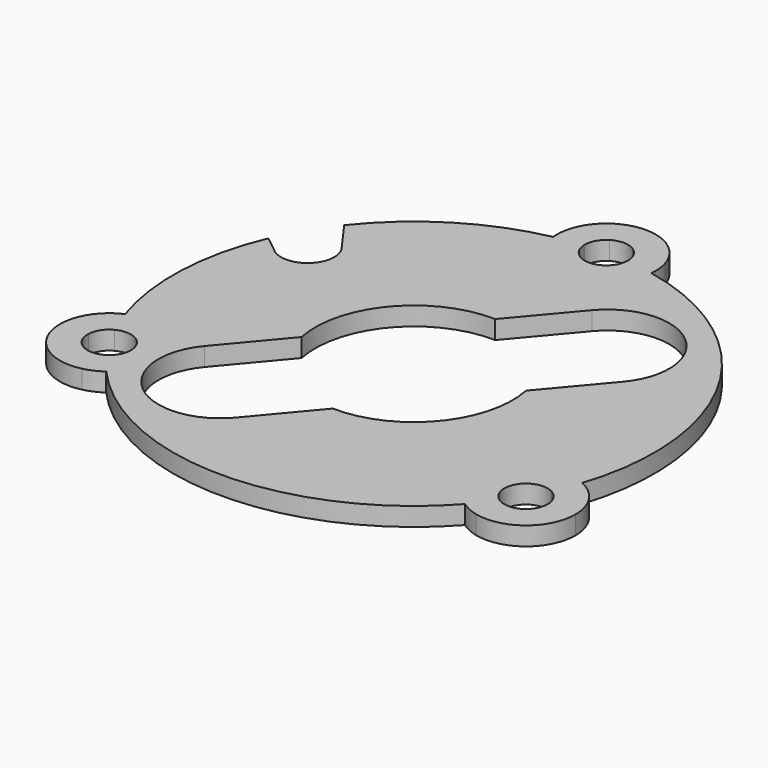
from build123d import *

# Parameters (mm, degrees)
F1_DEPTH = 1.5


# Not quite as in the source:
# - a feature names something its author has since deleted; it is built from what else it names


with BuildPart() as f1:
    # F0 (on Top) → F1 (new body)
    with BuildSketch(Plane.XY):
        with BuildLine():
            Line((-16.6795244343, 6.6792241971), (-17.9256127972, 7.6760931368))
            ThreePointArc((-17.9256127972, 7.6760931368), (-19.4817711686, 0.8429662711), (-18.5216556944, -6.0990384764))
            ThreePointArc((-18.5216556944, -6.0990384764), (-18.1379825879, -7.1598594707), (-17.6936088333, -8.1967192494))
            ThreePointArc((-17.6936088333, -8.1967192494), (-15.9787045712, -8.2544735786), (-15.1374953738, -9.75))
            ThreePointArc((-15.1374953738, -9.75), (-15.3526962413, -10.5907684717), (-15.9453715143, -11.2247551096))
            ThreePointArc((-15.9453715143, -11.2247551096), (-15.2696114831, -12.1280239592), (-14.5427501065, -12.9907051133))
            ThreePointArc((-14.5427501065, -12.9907051133), (0, -19.5), (14.5427501065, -12.9907051133))
            ThreePointArc((14.5427501065, -12.9907051133), (13.4233937587, -7.75), (18.5216556944, -6.0990384764))
            ThreePointArc((18.5216556944, -6.0990384764), (16.8874953738, 9.75), (3.978905588, 19.0897435897))
            ThreePointArc((3.978905588, 19.0897435897), (0, 15.5), (-3.978905588, 19.0897435897))
            ThreePointArc((-3.978905588, 19.0897435897), (-10.2620358256, 16.5813335023), (-15.3099476357, 12.0770651813))
            Line((-15.3099476357, 12.0770651813), (-13.4680928187, 9.5194474719))
            ThreePointArc((-13.4680928187, 9.5194474719), (-13.7890746093, 6.6466910805), (-16.6795244343, 6.6792241971))
        make_face()
        with BuildLine():
            ThreePointArc((4.2189837175, 12.7847634468), (11.2638316679, 13.3931361584), (11.8722043795, 6.348288208))
            Line((11.8722043795, 6.348288208), (7.846187435, 1.5611991336))
            ThreePointArc((7.846187435, 1.5611991336), (6.128355545, -5.1423008775), (-0.1750048611, -7.9980856021))
            Line((-0.1750048611, -7.9980856021), (-4.1902567902, -12.7942075969))
            ThreePointArc((-4.1902567902, -12.7942075969), (-11.2337204833, -13.4184024423), (-11.8579153287, -6.3749387493))
            Line((-11.8579153287, -6.3749387493), (-7.8426609809, -1.5788187794))
            ThreePointArc((-7.8426609809, -1.5788187794), (-6.128355545, 5.1423008775), (0.1929691871, 7.9976723422))
            Line((0.1929691871, 7.9976723422), (4.2189837175, 12.7847634468))
        make_face(mode=Mode.SUBTRACT)
        with BuildLine():
            ThreePointArc((-17.6936088333, -8.1967192494), (-18.1379825879, -7.1598594707), (-18.5216556944, -6.0990384764))
            ThreePointArc((-18.5216556944, -6.0990384764), (-19.2041408378, -6.4891483024), (-19.7971496554, -7.0052027467))
            ThreePointArc((-19.7971496554, -7.0052027467), (-19.2630878929, -8.3626218874), (-18.6360824437, -9.6796916868))
            ThreePointArc((-18.6360824437, -9.6796916868), (-18.36446034, -8.8113443184), (-17.6936088333, -8.1967192494))
        make_face()
        with BuildLine():
            ThreePointArc((-18.6360824437, -9.6796916868), (-19.2630878929, -8.3626218874), (-19.7971496554, -7.0052027467))
            ThreePointArc((-19.7971496554, -7.0052027467), (-20.3515969889, -11.75), (-15.965258365, -13.6422331507))
            ThreePointArc((-15.965258365, -13.6422331507), (-16.8737869432, -12.5010125269), (-17.7009001234, -11.2994749799))
            ThreePointArc((-17.7009001234, -11.2994749799), (-18.4030398304, -10.625), (-18.6360824437, -9.6796916868))
        make_face()
        with BuildLine():
            ThreePointArc((-14.5427501065, -12.9907051133), (-15.2696114831, -12.1280239592), (-15.9453715143, -11.2247551096))
            ThreePointArc((-15.9453715143, -11.2247551096), (-16.8130781912, -11.498417022), (-17.7009001234, -11.2994749799))
            ThreePointArc((-17.7009001234, -11.2994749799), (-16.8737869432, -12.5010125269), (-15.965258365, -13.6422331507))
            ThreePointArc((-15.965258365, -13.6422331507), (-15.2218376977, -13.3866996722), (-14.5427501065, -12.9907051133))
        make_face()
        with BuildLine():
            ThreePointArc((17.7009001234, -11.2994749799), (16.8737869432, -12.5010125269), (15.965258365, -13.6422331507))
            ThreePointArc((15.965258365, -13.6422331507), (19.3685286228, -12.8875904796), (20.8874953738, -9.75))
            ThreePointArc((20.8874953738, -9.75), (20.6049284348, -8.2732835625), (19.7971496554, -7.0052027467))
            ThreePointArc((19.7971496554, -7.0052027467), (19.2630878929, -8.3626218874), (18.6360824437, -9.6796916868))
            ThreePointArc((18.6360824437, -9.6796916868), (18.6371421056, -9.7148387455), (18.6374953738, -9.75))
            ThreePointArc((18.6374953738, -9.75), (18.3851532639, -10.6552739056), (17.7009001234, -11.2994749799))
        make_face()
        with BuildLine():
            ThreePointArc((14.5427501065, -12.9907051133), (15.2218376977, -13.3866996722), (15.965258365, -13.6422331507))
            ThreePointArc((15.965258365, -13.6422331507), (16.8737869432, -12.5010125269), (17.7009001234, -11.2994749799))
            ThreePointArc((17.7009001234, -11.2994749799), (16.8130781912, -11.498417022), (15.9453715143, -11.2247551096))
            ThreePointArc((15.9453715143, -11.2247551096), (15.2696114831, -12.1280239592), (14.5427501065, -12.9907051133))
        make_face()
        with BuildLine():
            ThreePointArc((-4, 19.5), (-3.994722916, 19.2946008177), (-3.978905588, 19.0897435897))
            ThreePointArc((-3.978905588, 19.0897435897), (-2.8683711048, 19.2878834299), (-1.748237319, 19.421474359))
            ThreePointArc((-1.748237319, 19.421474359), (-1.7495592743, 19.4607272889), (-1.75, 19.5))
            Line((-1.75, 19.5), (-4, 19.5))
        make_face()
        with BuildLine():
            ThreePointArc((-1.748237319, 19.421474359), (-2.8683711048, 19.2878834299), (-3.978905588, 19.0897435897))
            ThreePointArc((-3.978905588, 19.0897435897), (0, 15.5), (3.978905588, 19.0897435897))
            ThreePointArc((3.978905588, 19.0897435897), (2.8683711048, 19.2878834299), (1.748237319, 19.421474359))
            ThreePointArc((1.748237319, 19.421474359), (0, 17.75), (-1.748237319, 19.421474359))
        make_face()
        with BuildLine():
            ThreePointArc((18.5216556944, -6.0990384764), (13.4233937587, -7.75), (14.5427501065, -12.9907051133))
            ThreePointArc((14.5427501065, -12.9907051133), (15.2696114831, -12.1280239592), (15.9453715143, -11.2247551096))
            ThreePointArc((15.9453715143, -11.2247551096), (15.3719509172, -8.875), (17.6936088333, -8.1967192493))
            ThreePointArc((17.6936088333, -8.1967192493), (18.1379825879, -7.1598594707), (18.5216556944, -6.0990384764))
        make_face()
        with BuildLine():
            ThreePointArc((-3.8318912904, 20.6474358974), (-3.9577496865, 20.0798425814), (-4, 19.5))
            Line((-4, 19.5), (-1.75, 19.5))
            ThreePointArc((-1.75, 19.5), (-1.5328191447, 20.3443728263), (-0.9351823203, 20.9791666667))
            ThreePointArc((-0.9351823203, 20.9791666667), (-2.3893009497, 20.8636344143), (-3.8318912904, 20.6474358974))
        make_face()
        with BuildLine():
            ThreePointArc((1.748237319, 19.421474359), (2.8683711048, 19.2878834299), (3.978905588, 19.0897435897))
            ThreePointArc((3.978905588, 19.0897435897), (3.994722916, 19.2946008177), (4, 19.5))
            Line((4, 19.5), (1.75, 19.5))
            ThreePointArc((1.75, 19.5), (1.7495592743, 19.4607272889), (1.748237319, 19.421474359))
        make_face()
        with BuildLine():
            ThreePointArc((3.8318912904, 20.6474358974), (0, 23.5), (-3.8318912904, 20.6474358974))
            ThreePointArc((-3.8318912904, 20.6474358974), (-2.3893009497, 20.8636344143), (-0.9351823203, 20.9791666667))
            ThreePointArc((-0.9351823203, 20.9791666667), (0, 21.25), (0.9351823203, 20.9791666667))
            ThreePointArc((0.9351823203, 20.9791666667), (2.3893009497, 20.8636344143), (3.8318912904, 20.6474358974))
        make_face()
        with BuildLine():
            ThreePointArc((19.7971496554, -7.0052027467), (19.2041408378, -6.4891483024), (18.5216556944, -6.0990384764))
            ThreePointArc((18.5216556944, -6.0990384764), (18.1379825879, -7.1598594707), (17.6936088333, -8.1967192493))
            ThreePointArc((17.6936088333, -8.1967192493), (18.36446034, -8.8113443184), (18.6360824437, -9.6796916868))
            ThreePointArc((18.6360824437, -9.6796916868), (19.2630878929, -8.3626218874), (19.7971496554, -7.0052027467))
        make_face()
        with BuildLine():
            Line((1.75, 19.5), (4, 19.5))
            ThreePointArc((4, 19.5), (3.9577496865, 20.0798425814), (3.8318912904, 20.6474358974))
            ThreePointArc((3.8318912904, 20.6474358974), (2.3893009497, 20.8636344143), (0.9351823203, 20.9791666667))
            ThreePointArc((0.9351823203, 20.9791666667), (1.5328191447, 20.3443728263), (1.75, 19.5))
        make_face()
    extrude(amount=F1_DEPTH)


solid = f1.part
